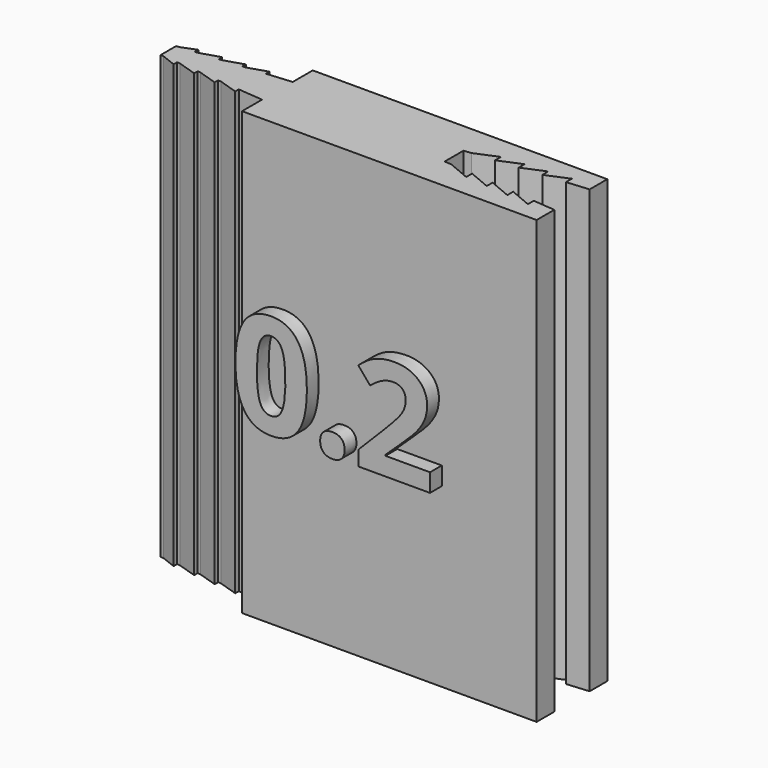
from build123d import *

# Parameters (mm, degrees)
F1_DEPTH     = 30
F2_TEXT_SIZE = 9.7222222222
F3_DEPTH     = 1


# Not quite as in the source:
# - Text() gives the source's letters only with a copy of the font that has no kerning and outlines rounded to 1/6400 em; it was checked with that copy


with BuildPart() as f1:
    # F0 (on Top) → F1 (new body)
    with BuildSketch(Plane.XY):
        Polygon((-10, -3), (10, -3), (10, -1.5), (8.5, -1.3687670047), (8.5, -1.8687670047), (7, -1.2375340094), (7, -1.7375340094), (5.5, -1.1063010141), (5.5, -1.6063010141), (4, -0.9750680188), (4, -1.4750680188), (2.5, -0.8438350236), (2, -0.8000906918), (2, 0), (2, 0.8000906918), (2.5, 0.8438350236), (4, 1.4750680188), (4, 0.9750680188), (5.5, 1.6063010141), (5.5, 1.1063010141), (7, 1.7375340094), (7, 1.2375340094), (8.5, 1.8687670047), (8.5, 1.3687670047), (10, 1.5), (10, 3), (-10, 3), (-10, 1.3), (-11.7, 1.151269272), (-11.7, 1.451269272), (-13, 1.0375340094), (-13.2, 1.0200362767), (-13.2, 1.3200362767), (-14.5, 0.9063010141), (-14.7, 0.8888032814), (-14.7, 1.1888032814), (-16, 0.7750680188), (-16.2, 0.7575702861), (-16.2, 1.0575702861), (-17.2007610604, 0.6700150385), (-17.4, 0.6525838899), (-17.4, 0), (-17.4, -0.6525838899), (-17.2007610604, -0.6700150385), (-16.2, -1.0575702861), (-16.2, -0.7575702861), (-16, -0.7750680188), (-14.7, -1.1888032814), (-14.7, -0.8888032814), (-14.5, -0.9063010141), (-13.2, -1.3200362767), (-13.2, -1.0200362767), (-13, -1.0375340094), (-11.7, -1.451269272), (-11.7, -1.151269272), (-10, -1.3), align=None)
    extrude(amount=F1_DEPTH)

    # F2 (on face) → F3 (join)
    with BuildSketch(Plane.XZ.offset(3)):
        with Locations((-10, 12)):
            Text('0.2', F2_TEXT_SIZE, font='Open Sans', font_style=FontStyle.BOLD, text_align=(TextAlign.LEFT, TextAlign.BOTTOM))
    extrude(amount=F3_DEPTH)


solid = f1.part
